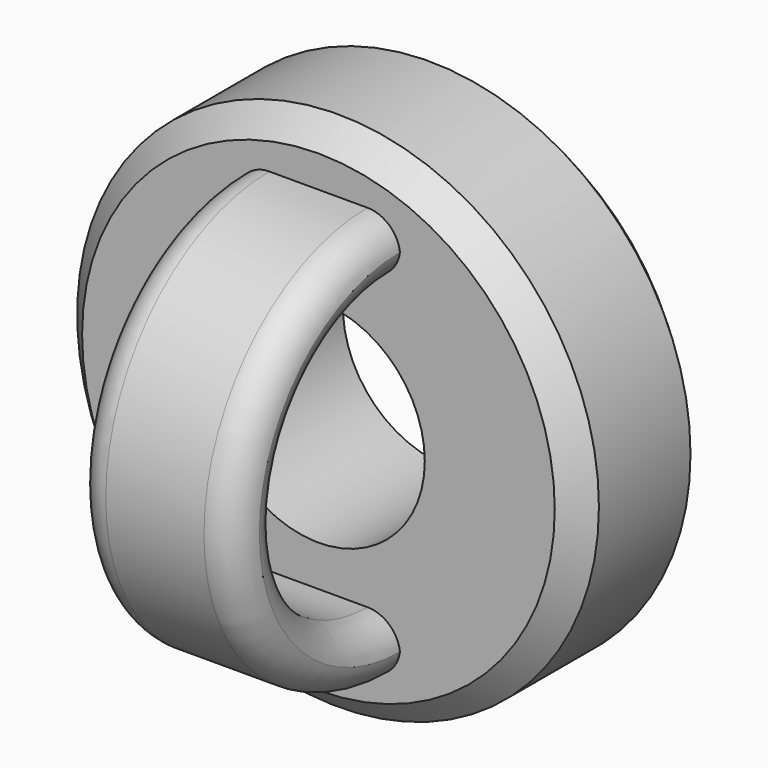
from build123d import *

# Parameters (mm, degrees)
F0_R        = 40.5136792868
F0_R_2      = 16.5163542796
F1_DEPTH    = 25.4
F2_W        = 25.4
F2_H        = 8.89
F3_ANGLE    = 180
F4_T2_ANGLE = 180
F4_T4_ANGLE = 180
F4_T6_ANGLE = 180
F5_SIZE     = 3.81


# Not quite as in the source:
# - a fillet or chamfer that OpenCascade refuses, or shapes differently, is made with other operations: its cross-section is extruded or revolved along the edge and cut away or added


with BuildPart() as f1:
    # F0 (on Front) → F1 (new body)
    with BuildSketch(Plane.XZ):
        Circle(F0_R)
        Circle(F0_R_2, mode=Mode.SUBTRACT)
    extrude(amount=F1_DEPTH)

    # F2 (on face) → F3 (revolve)
    with BuildSketch(Plane.XZ.offset(25.4)):
        with Locations((0, 27.305)):
            Rectangle(F2_W, F2_H)
    revolve(axis=Axis((-4.5374315232, -25.4, 0), (1, 0, 0)), revolution_arc=F3_ANGLE)

    # F4: fillet of radius 5.08 on 3 edges, made by hand

    # F4_s1 → F4_t2 (revolve, cut)
    with BuildSketch(Plane.XZ.offset(25.4)):
        with BuildLine():
            ThreePointArc((12.7, 27.94), (11.2121024484, 24.3478975516), (7.62, 22.86))
            Line((7.62, 22.86), (12.7, 22.86))
            Line((12.7, 22.86), (12.7, 27.94))
        make_face()
    revolve(axis=Axis((12.7, -25.4, 0), (1, 0, 0)), revolution_arc=F4_T2_ANGLE, mode=Mode.SUBTRACT)

    # F4_s3 → F4_t4 (revolve, cut)
    with BuildSketch(Plane.XZ.offset(25.4)):
        with BuildLine():
            ThreePointArc((12.7, 26.67), (11.2121024484, 30.2621024484), (7.62, 31.75))
            Line((7.62, 31.75), (12.7, 31.75))
            Line((12.7, 31.75), (12.7, 26.67))
        make_face()
    revolve(axis=Axis((12.7, -25.4, 0), (1, 0, 0)), revolution_arc=F4_T4_ANGLE, mode=Mode.SUBTRACT)

    # F4_s5 → F4_t6 (revolve, cut)
    with BuildSketch(Plane.XZ.offset(25.4)):
        with BuildLine():
            ThreePointArc((-12.7, 26.67), (-11.2121024484, 30.2621024484), (-7.62, 31.75))
            Line((-7.62, 31.75), (-12.7, 31.75))
            Line((-12.7, 31.75), (-12.7, 26.67))
        make_face()
    revolve(axis=Axis((-12.7, -25.4, 0), (1, 0, 0)), revolution_arc=F4_T6_ANGLE, mode=Mode.SUBTRACT)

    # F5
    f5_edges = [f1.edges().sort_by_distance(p)[0] for p in [
        (-40.513679, -25.4, 0),
        (-40.513679, 0, 0),
    ]]
    chamfer(f5_edges, length=F5_SIZE)


solid = f1.part
